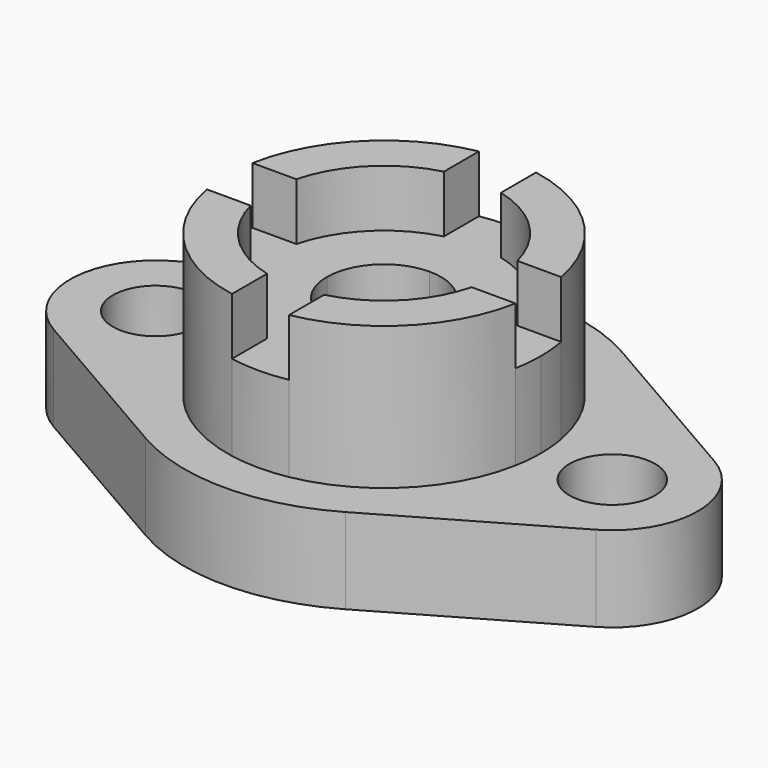
from build123d import *

# Parameters (mm, degrees)
F0_R     = 9.525
F1_DEPTH = 19.05
F2_DEPTH = 50.8
F3_DEPTH = 38.1


with BuildPart() as f1:
    # F0 (on Top) → F1 (new body)
    with BuildSketch(Plane.XY):
        with BuildLine():
            Line((-60.325, -16.4977839421), (-22.225, -38.4948291982))
            ThreePointArc((-22.225, -38.4948291982), (0, -44.45), (22.225, -38.4948291982))
            Line((22.225, -38.4948291982), (60.325, -16.4977839421))
            ThreePointArc((60.325, -16.4977839421), (69.85, 0), (60.325, 16.4977839421))
            Line((60.325, 16.4977839421), (22.225, 38.4948291982))
            ThreePointArc((22.225, 38.4948291982), (0, 44.45), (-22.225, 38.4948291982))
            Line((-22.225, 38.4948291982), (-60.325, 16.4977839421))
            ThreePointArc((-60.325, 16.4977839421), (-69.85, 0), (-60.325, -16.4977839421))
        make_face()
        with Locations((-50.8, 0)):
            Circle(F0_R, mode=Mode.SUBTRACT)
        with BuildLine():
            ThreePointArc((6.35, 34.3428758988), (24.6957043329, 24.6957043329), (34.3428758988, 6.35))
            ThreePointArc((34.3428758988, 6.35), (34.7791644937, 3.1883133656), (34.925, 0))
            ThreePointArc((34.925, 0), (34.7791644937, -3.1883133656), (34.3428758988, -6.35))
            ThreePointArc((34.3428758988, -6.35), (24.6957043329, -24.6957043329), (6.35, -34.3428758988))
            ThreePointArc((6.35, -34.3428758988), (0, -34.925), (-6.35, -34.3428758988))
            ThreePointArc((-6.35, -34.3428758988), (-24.6957043329, -24.6957043329), (-34.3428758988, -6.35))
            ThreePointArc((-34.3428758988, -6.35), (-34.925, 0), (-34.3428758988, 6.35))
            ThreePointArc((-34.3428758988, 6.35), (-24.6957043329, 24.6957043329), (-6.35, 34.3428758988))
            ThreePointArc((-6.35, 34.3428758988), (0, 34.925), (6.35, 34.3428758988))
        make_face(mode=Mode.SUBTRACT)
        with Locations((50.8, 0)):
            Circle(F0_R, mode=Mode.SUBTRACT)
    extrude(amount=F1_DEPTH)

    # F0 (on Top) → F2 (join)
    with BuildSketch(Plane.XY):
        with BuildLine():
            ThreePointArc((-24.5934442484, 6.35), (-17.9605122421, 17.9605122421), (-6.35, 24.5934442484))
            Line((-6.35, 24.5934442484), (-6.35, 34.3428758988))
            ThreePointArc((-6.35, 34.3428758988), (-24.6957043329, 24.6957043329), (-34.3428758988, 6.35))
            Line((-34.3428758988, 6.35), (-30.5676609278, 6.35))
            Line((-30.5676609278, 6.35), (-24.5934442484, 6.35))
        make_face()
        with BuildLine():
            Line((-6.35, -34.3428758988), (-6.35, -24.5934442484))
            ThreePointArc((-6.35, -24.5934442484), (-17.9605122421, -17.9605122421), (-24.5934442484, -6.35))
            Line((-24.5934442484, -6.35), (-34.3428758988, -6.35))
            ThreePointArc((-34.3428758988, -6.35), (-24.6957043329, -24.6957043329), (-6.35, -34.3428758988))
        make_face()
        with BuildLine():
            Line((25.4, -6.35), (24.5934442484, -6.35))
            ThreePointArc((24.5934442484, -6.35), (17.9605122421, -17.9605122421), (6.35, -24.5934442484))
            Line((6.35, -24.5934442484), (6.35, -29.9044754356))
            Line((6.35, -29.9044754356), (6.35, -34.3428758988))
            ThreePointArc((6.35, -34.3428758988), (24.6957043329, -24.6957043329), (34.3428758988, -6.35))
            Line((34.3428758988, -6.35), (25.4, -6.35))
        make_face()
        with BuildLine():
            ThreePointArc((6.35, 24.5934442484), (17.9605122421, 17.9605122421), (24.5934442484, 6.35))
            Line((24.5934442484, 6.35), (34.3428758988, 6.35))
            ThreePointArc((34.3428758988, 6.35), (24.6957043329, 24.6957043329), (6.35, 34.3428758988))
            Line((6.35, 34.3428758988), (6.35, 25.4))
            Line((6.35, 25.4), (6.35, 24.5934442484))
        make_face()
    extrude(amount=F2_DEPTH)

    # F0 (on Top) → F3 (join)
    with BuildSketch(Plane.XY):
        with BuildLine():
            ThreePointArc((24.5934442484, -6.35), (25.1975542852, -3.2005090291), (25.4, 0))
            ThreePointArc((25.4, 0), (25.1975542852, 3.2005090291), (24.5934442484, 6.35))
            ThreePointArc((24.5934442484, 6.35), (17.9605122421, 17.9605122421), (6.35, 24.5934442484))
            ThreePointArc((6.35, 24.5934442484), (0, 25.4), (-6.35, 24.5934442484))
            ThreePointArc((-6.35, 24.5934442484), (-17.9605122421, 17.9605122421), (-24.5934442484, 6.35))
            ThreePointArc((-24.5934442484, 6.35), (-25.4, 0), (-24.5934442484, -6.35))
            ThreePointArc((-24.5934442484, -6.35), (-17.9605122421, -17.9605122421), (-6.35, -24.5934442484))
            ThreePointArc((-6.35, -24.5934442484), (0, -25.4), (6.35, -24.5934442484))
            ThreePointArc((6.35, -24.5934442484), (17.9605122421, -17.9605122421), (24.5934442484, -6.35))
        make_face()
        with BuildLine():
            ThreePointArc((0, 12.7), (8.9802561211, 8.9802561211), (12.7, 0))
            ThreePointArc((12.7, 0), (8.9802561211, -8.9802561211), (0, -12.7))
            ThreePointArc((0, -12.7), (-8.9802561211, -8.9802561211), (-12.7, 0))
            ThreePointArc((-12.7, 0), (-8.9802561211, 8.9802561211), (0, 12.7))
        make_face(mode=Mode.SUBTRACT)
        with BuildLine():
            ThreePointArc((24.5934442484, 6.35), (25.1975542852, 3.2005090291), (25.4, 0))
            ThreePointArc((25.4, 0), (25.1975542852, -3.2005090291), (24.5934442484, -6.35))
            Line((24.5934442484, -6.35), (25.4, -6.35))
            Line((25.4, -6.35), (34.3428758988, -6.35))
            ThreePointArc((34.3428758988, -6.35), (34.7791644937, -3.1883133656), (34.925, 0))
            ThreePointArc((34.925, 0), (34.7791644937, 3.1883133656), (34.3428758988, 6.35))
            Line((34.3428758988, 6.35), (24.5934442484, 6.35))
        make_face()
        with BuildLine():
            ThreePointArc((-6.35, 24.5934442484), (0, 25.4), (6.35, 24.5934442484))
            Line((6.35, 24.5934442484), (6.35, 25.4))
            Line((6.35, 25.4), (6.35, 34.3428758988))
            ThreePointArc((6.35, 34.3428758988), (0, 34.925), (-6.35, 34.3428758988))
            Line((-6.35, 34.3428758988), (-6.35, 24.5934442484))
        make_face()
        with BuildLine():
            Line((6.35, -29.9044754356), (6.35, -24.5934442484))
            ThreePointArc((6.35, -24.5934442484), (0, -25.4), (-6.35, -24.5934442484))
            Line((-6.35, -24.5934442484), (-6.35, -34.3428758988))
            ThreePointArc((-6.35, -34.3428758988), (0, -34.925), (6.35, -34.3428758988))
            Line((6.35, -34.3428758988), (6.35, -29.9044754356))
        make_face()
        with BuildLine():
            ThreePointArc((-24.5934442484, -6.35), (-25.4, 0), (-24.5934442484, 6.35))
            Line((-24.5934442484, 6.35), (-30.5676609278, 6.35))
            Line((-30.5676609278, 6.35), (-34.3428758988, 6.35))
            ThreePointArc((-34.3428758988, 6.35), (-34.925, 0), (-34.3428758988, -6.35))
            Line((-34.3428758988, -6.35), (-24.5934442484, -6.35))
        make_face()
    extrude(amount=F3_DEPTH)


solid = f1.part
